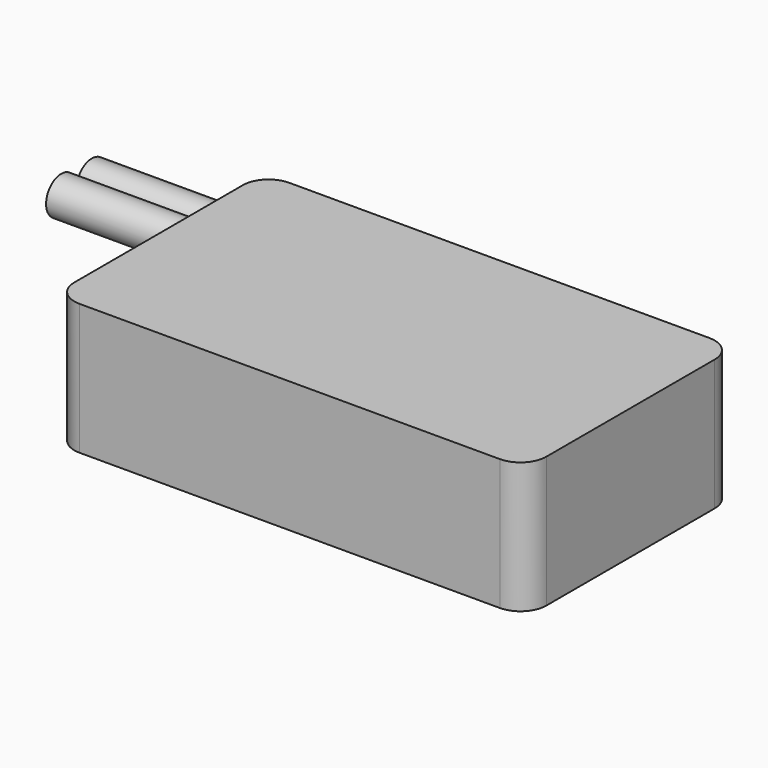
from build123d import *

# Parameters (mm, degrees)
F0_W         = 91.44
F0_H         = 50.8
F1_DEPTH     = 25.4
F2_R         = 5
F4_R         = 3.7455857162
F5_DEPTH     = 25
F4_R_2       = 3.6615290914
F6_DEPTH     = 25
F7_TEXT_SIZE = 14.7047043701
F8_DEPTH     = 10.16


# Not quite as in the source:
# - Text() gives the source's letters only with a copy of the font that has no kerning and outlines rounded to 1/6400 em; it was checked with that copy


with BuildPart() as f1:
    # F0 (on Top) → F1 (new body)
    with BuildSketch(Plane.XY):
        Rectangle(F0_W, F0_H)
    extrude(amount=-F1_DEPTH)

    # F2
    f2_edges = [f1.edges().sort_by_distance(p)[0] for p in [
        (45.72, -25.4, -12.7),
        (-45.72, -25.4, -12.7),
        (45.72, 25.4, -12.7),
        (-45.72, 25.4, -12.7),
    ]]
    fillet(f2_edges, radius=F2_R)

    # F4 (on face) → F5 (join)
    with BuildSketch(Plane(origin=(-45.72, 0, 0), x_dir=(0, -1, 0), z_dir=(-1, 0, 0))):
        with Locations((-15.0797893293, -5.1476373337)):
            Circle(F4_R)
    extrude(amount=F5_DEPTH)

    # F4 (on face) → F6 (join)
    with BuildSketch(Plane(origin=(-45.72, 0, 0), x_dir=(0, -1, 0), z_dir=(-1, 0, 0))):
        with Locations((-15.0797893293, -5.1476373337)):
            Circle(F4_R)
        with Locations((-7.6595754363, -4.6689137816)):
            Circle(F4_R_2)
    extrude(amount=F6_DEPTH)

    # F7 (on face) → F8 (cut)
    with BuildSketch(Plane(origin=(0, 0, -25.4), x_dir=(1, 0, 0), z_dir=(0, 0, -1))):
        with Locations((-45.72, 0)):
            Text('Lipo Battery', F7_TEXT_SIZE, font='Open Sans', text_align=(TextAlign.LEFT, TextAlign.BOTTOM))
    extrude(amount=-F8_DEPTH, mode=Mode.SUBTRACT)


solid = f1.part
